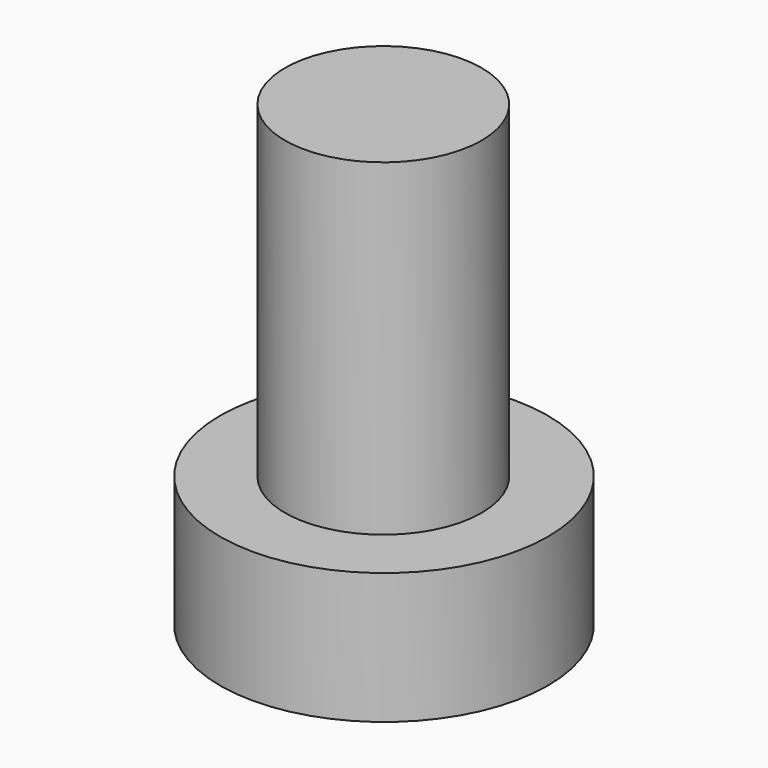
from build123d import *

# Parameters (mm, degrees)
F0_R     = 1.5
F1_DEPTH = 5
F2_R     = 2.5
F2_R_2   = 1.5
F3_DEPTH = 2


with BuildPart() as f1:
    # F0 (on Top) → F1 (new body)
    with BuildSketch(Plane.XY):
        Circle(F0_R)
    extrude(amount=F1_DEPTH)

    # F2 (on face) → F3 (join)
    with BuildSketch(Plane(origin=(0, 0, 0), x_dir=(1, 0, 0), z_dir=(0, 0, -1))):
        with Locations((0, -0.0132801069)):
            Circle(F2_R)
        Circle(F2_R_2, mode=Mode.SUBTRACT)
        Circle(F2_R_2)
    extrude(amount=F3_DEPTH)


solid = f1.part
